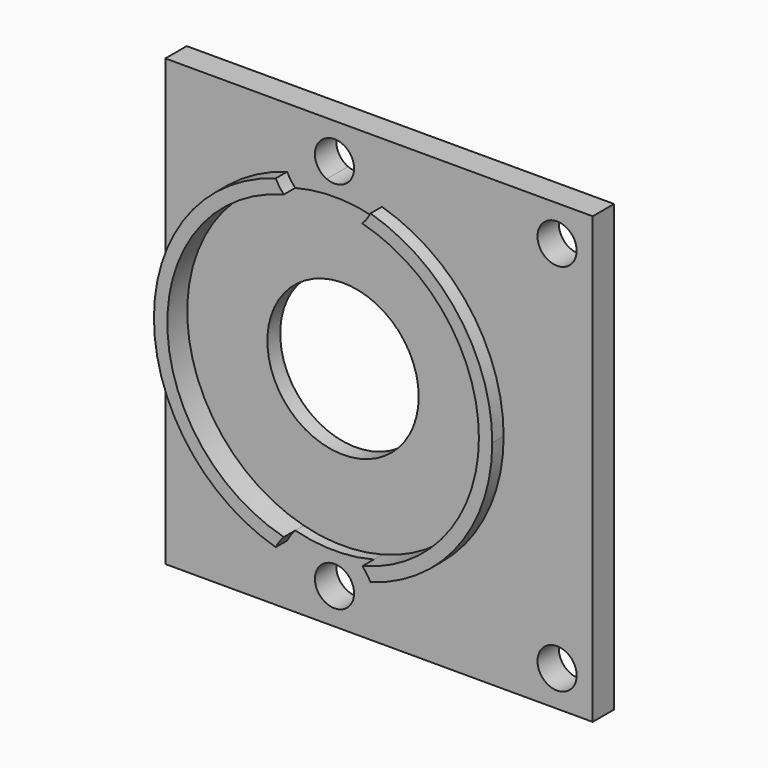
from build123d import *

# Parameters (mm, degrees)
F1_DEPTH = 1.5
F0_R     = 1.1
F2_DEPTH = 1.5
F3_DEPTH = 2.3
F0_R_2   = 4.25
F4_DEPTH = 0.9


with BuildPart() as f1:
    # F0 (on Front) → F1 (new body)
    with BuildSketch(Plane.XZ):
        with BuildLine():
            Line((-4.7360679775, 12.5), (-12, 12.5))
            Line((-12, 12.5), (-12, 0))
            ThreePointArc((-12, 0), (-10.101019661, 5.6986401986), (-5.1632631341, 9.119047619))
            ThreePointArc((-5.1632631341, 9.119047619), (-5.476335177, 10.8760703579), (-4.7360679775, 12.5))
        make_face()
    extrude(amount=F1_DEPTH)



with BuildPart() as f1b:
    # F0 (on Front) → F1, piece 2 (new body)
    with BuildSketch(Plane.XZ):
        with BuildLine():
            ThreePointArc((-5.1632631341, -9.119047619), (-10.101019661, -5.6986401986), (-12, 0))
            Line((-12, 0), (-12, -12.5))
            Line((-12, -12.5), (-4.7360679775, -12.5))
            ThreePointArc((-4.7360679775, -12.5), (-5.476335177, -10.8760703579), (-5.1632631341, -9.119047619))
        make_face()
    extrude(amount=F1_DEPTH)


with BuildPart() as f1c:
    # F0 (on Front) → F1, piece 3 (new body)
    with BuildSketch(Plane.XZ):
        with BuildLine():
            Line((12, 12.5), (-0.2639320225, 12.5))
            ThreePointArc((-0.2639320225, 12.5), (0.3025170769, 11.5704662693), (0.5, 10.5))
            ThreePointArc((0.5, 10.5), (0.4146002644, 9.7892923957), (0.1632631341, 9.119047619))
            ThreePointArc((0.1632631341, 9.119047619), (5.101019661, 5.6986401986), (7, 0))
            ThreePointArc((7, 0), (5.101019661, -5.6986401986), (0.1632631341, -9.119047619))
            ThreePointArc((0.1632631341, -9.119047619), (0.4146002644, -9.7892923957), (0.5, -10.5))
            ThreePointArc((0.5, -10.5), (0.3025170769, -11.5704662693), (-0.2639320225, -12.5))
            Line((-0.2639320225, -12.5), (12, -12.5))
            Line((12, -12.5), (12, 12.5))
        make_face()
        with Locations((10, -10.5)):
            Circle(F0_R, mode=Mode.SUBTRACT)
        with Locations((10, 10.5)):
            Circle(F0_R, mode=Mode.SUBTRACT)
    extrude(amount=F1_DEPTH)


with BuildPart() as f1d:
    # F0 (on Front) → F1, piece 4 (new body)
    with BuildSketch(Plane.XZ):
        with BuildLine():
            ThreePointArc((-2.9357751714, 9.49), (-4.0605803478, 9.370943868), (-5.1632631341, 9.119047619))
            ThreePointArc((-5.1632631341, 9.119047619), (-4.956519224, 8.7779334211), (-4.7063489833, 8.4672619048))
            ThreePointArc((-4.7063489833, 8.4672619048), (-2.5, 8.75), (-0.2936510167, 8.4672619048))
            ThreePointArc((-0.2936510167, 8.4672619048), (-0.043480776, 8.7779334211), (0.1632631341, 9.119047619))
            ThreePointArc((0.1632631341, 9.119047619), (-0.9394196522, 9.370943868), (-2.0642248286, 9.49))
            ThreePointArc((-2.0642248286, 9.49), (-2.5, 9.4), (-2.9357751714, 9.49))
        make_face()
    extrude(amount=F1_DEPTH)


with BuildPart() as f1_1:
    add(f1.part)

    add(f1b.part)  # F2 merges F1b

    add(f1c.part)  # F2 merges F1c

    add(f1d.part)  # F2 merges F1d
    # F0 (on Front) → F2 (join)
    with BuildSketch(Plane.XZ):
        with BuildLine():
            Line((12, 12.5), (-0.2639320225, 12.5))
            ThreePointArc((-0.2639320225, 12.5), (0.3025170769, 11.5704662693), (0.5, 10.5))
            ThreePointArc((0.5, 10.5), (0.4146002644, 9.7892923957), (0.1632631341, 9.119047619))
            ThreePointArc((0.1632631341, 9.119047619), (5.101019661, 5.6986401986), (7, 0))
            ThreePointArc((7, 0), (5.101019661, -5.6986401986), (0.1632631341, -9.119047619))
            ThreePointArc((0.1632631341, -9.119047619), (0.4146002644, -9.7892923957), (0.5, -10.5))
            ThreePointArc((0.5, -10.5), (0.3025170769, -11.5704662693), (-0.2639320225, -12.5))
            Line((-0.2639320225, -12.5), (12, -12.5))
            Line((12, -12.5), (12, 12.5))
        make_face()
        with Locations((10, -10.5)):
            Circle(F0_R, mode=Mode.SUBTRACT)
        with Locations((10, 10.5)):
            Circle(F0_R, mode=Mode.SUBTRACT)
        with BuildLine():
            ThreePointArc((-2.9357751714, -9.49), (-4.0605803478, -9.370943868), (-5.1632631341, -9.119047619))
            ThreePointArc((-5.1632631341, -9.119047619), (-5.476335177, -10.8760703579), (-4.7360679775, -12.5))
            Line((-4.7360679775, -12.5), (-0.2639320225, -12.5))
            ThreePointArc((-0.2639320225, -12.5), (0.3025170769, -11.5704662693), (0.5, -10.5))
            ThreePointArc((0.5, -10.5), (0.4146002644, -9.7892923957), (0.1632631341, -9.119047619))
            ThreePointArc((0.1632631341, -9.119047619), (-0.9394196522, -9.370943868), (-2.0642248286, -9.49))
            ThreePointArc((-2.0642248286, -9.49), (-1.5809372468, -9.8955799013), (-1.4, -10.5))
            ThreePointArc((-1.4, -10.5), (-3.1044200987, -11.4190627532), (-2.9357751714, -9.49))
        make_face()
        with BuildLine():
            Line((-0.2639320225, 12.5), (-4.7360679775, 12.5))
            ThreePointArc((-4.7360679775, 12.5), (-5.476335177, 10.8760703579), (-5.1632631341, 9.119047619))
            ThreePointArc((-5.1632631341, 9.119047619), (-4.0605803478, 9.370943868), (-2.9357751714, 9.49))
            ThreePointArc((-2.9357751714, 9.49), (-3.1044200987, 11.4190627532), (-1.4, 10.5))
            ThreePointArc((-1.4, 10.5), (-1.5809372468, 9.8955799013), (-2.0642248286, 9.49))
            ThreePointArc((-2.0642248286, 9.49), (-0.9394196522, 9.370943868), (0.1632631341, 9.119047619))
            ThreePointArc((0.1632631341, 9.119047619), (0.4146002644, 9.7892923957), (0.5, 10.5))
            ThreePointArc((0.5, 10.5), (0.3025170769, 11.5704662693), (-0.2639320225, 12.5))
        make_face()
        with BuildLine():
            ThreePointArc((-4.7063489833, -8.4672619048), (-4.956519224, -8.7779334211), (-5.1632631341, -9.119047619))
            ThreePointArc((-5.1632631341, -9.119047619), (-4.0605803478, -9.370943868), (-2.9357751714, -9.49))
            ThreePointArc((-2.9357751714, -9.49), (-2.5, -9.4), (-2.0642248286, -9.49))
            ThreePointArc((-2.0642248286, -9.49), (-0.9394196522, -9.370943868), (0.1632631341, -9.119047619))
            ThreePointArc((0.1632631341, -9.119047619), (-0.043480776, -8.7779334211), (-0.2936510167, -8.4672619048))
            ThreePointArc((-0.2936510167, -8.4672619048), (-2.5, -8.75), (-4.7063489833, -8.4672619048))
        make_face()
    extrude(amount=F2_DEPTH)

    # F0 (on Front) → F3 (join)
    with BuildSketch(Plane.XZ):
        with BuildLine():
            ThreePointArc((-5.1632631341, 9.119047619), (-10.101019661, 5.6986401986), (-12, 0))
            ThreePointArc((-12, 0), (-10.101019661, -5.6986401986), (-5.1632631341, -9.119047619))
            ThreePointArc((-5.1632631341, -9.119047619), (-4.956519224, -8.7779334211), (-4.7063489833, -8.4672619048))
            ThreePointArc((-4.7063489833, -8.4672619048), (-11.25, 0), (-4.7063489833, 8.4672619048))
            ThreePointArc((-4.7063489833, 8.4672619048), (-4.956519224, 8.7779334211), (-5.1632631341, 9.119047619))
        make_face()
        with BuildLine():
            ThreePointArc((7, 0), (5.101019661, 5.6986401986), (0.1632631341, 9.119047619))
            ThreePointArc((0.1632631341, 9.119047619), (-0.043480776, 8.7779334211), (-0.2936510167, 8.4672619048))
            ThreePointArc((-0.2936510167, 8.4672619048), (4.4234403877, 5.3505582137), (6.25, 0))
            ThreePointArc((6.25, 0), (4.4234403877, -5.3505582137), (-0.2936510167, -8.4672619048))
            ThreePointArc((-0.2936510167, -8.4672619048), (-0.043480776, -8.7779334211), (0.1632631341, -9.119047619))
            ThreePointArc((0.1632631341, -9.119047619), (5.101019661, -5.6986401986), (7, 0))
        make_face()
    extrude(amount=F3_DEPTH)

    # F0 (on Front) → F4 (join)
    with BuildSketch(Plane.XZ):
        with BuildLine():
            ThreePointArc((-0.2936510167, 8.4672619048), (-2.5, 7.5), (-4.7063489833, 8.4672619048))
            ThreePointArc((-4.7063489833, 8.4672619048), (-11.25, 0), (-4.7063489833, -8.4672619048))
            ThreePointArc((-4.7063489833, -8.4672619048), (-2.5, -7.5), (-0.2936510167, -8.4672619048))
            ThreePointArc((-0.2936510167, -8.4672619048), (4.4234403877, -5.3505582137), (6.25, 0))
            ThreePointArc((6.25, 0), (4.4234403877, 5.3505582137), (-0.2936510167, 8.4672619048))
        make_face()
        with Locations((-2.5, 0)):
            Circle(F0_R_2, mode=Mode.SUBTRACT)
        with BuildLine():
            ThreePointArc((-0.2936510167, 8.4672619048), (-2.5, 8.75), (-4.7063489833, 8.4672619048))
            ThreePointArc((-4.7063489833, 8.4672619048), (-2.5, 7.5), (-0.2936510167, 8.4672619048))
        make_face()
        with BuildLine():
            ThreePointArc((-0.2936510167, -8.4672619048), (-2.5, -7.5), (-4.7063489833, -8.4672619048))
            ThreePointArc((-4.7063489833, -8.4672619048), (-2.5, -8.75), (-0.2936510167, -8.4672619048))
        make_face()
    extrude(amount=F4_DEPTH)


solid = f1_1.part
